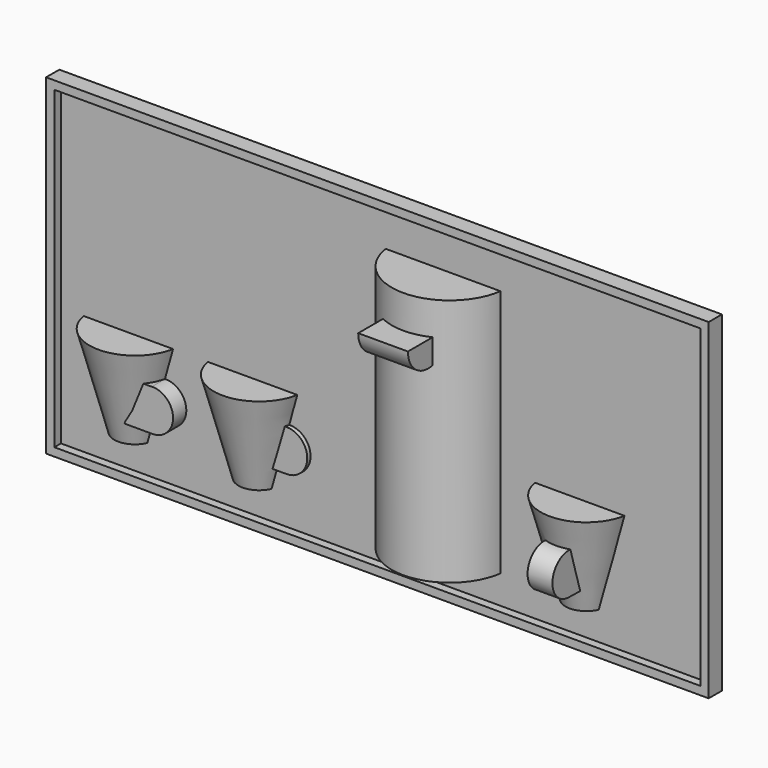
from build123d import *

# Parameters (mm, degrees)
F1_R      = 70
F2_DEPTH  = 300
F3_R      = 25
F4_R      = 55
F6_R      = 25
F7_R      = 55
F9_R      = 25
F10_R     = 55
F14_DEPTH = 30
F17_DEPTH = 15
F19_DEPTH = 15
F21_DEPTH = 30
F22_W     = 800
F22_H     = 400
F24_DEPTH = 20
F25_T     = -10


# Not quite as in the source:
# - a feature names something its author has since deleted; it is built from what else it names


with BuildPart() as f2:
    # F1 (on Top) → F2 (new body)
    with BuildSketch(Plane.XY):
        with Locations((70, 0)):
            Circle(F1_R)
    extrude(amount=F2_DEPTH)

    # F13 (on offset) → F14 (join, symmetric)
    with BuildSketch(Plane.YZ.offset(70)):
        with BuildLine():
            Line((-39.4232119037, 259.9333557068), (-100.5767880963, 259.9333557068))
            ThreePointArc((-100.5767880963, 259.9333557068), (-70, 229.4231392758), (-39.4232119037, 259.9333557068))
        make_face()
    extrude(amount=F14_DEPTH, both=True)


with BuildPart() as f5:
    # F3 (on Top) → F5 section 0
    with BuildSketch(Plane.XY):
        with Locations((235, 0)):
            Circle(F3_R)
    # F4 (on offset) → F5 section 1
    with BuildSketch(Plane.XY.offset(110)):
        with Locations((235, 0)):
            Circle(F4_R)
    loft()

    # F16 (on offset) → F17 (join, symmetric)
    with BuildSketch(Plane.YZ.offset(235)):
        with BuildLine():
            Line((-13.6413012409, 73.7935081125), (-44.023681798, 74.9809287811))
            ThreePointArc((-44.023681798, 74.9809287811), (-69.9889457828, 50.7433630762), (-45.5103433285, 25.005209549))
            Line((-45.5103433285, 25.005209549), (-13.6413012409, 24.3545078339))
            Line((-13.6413012409, 24.3545078339), (-13.6413012409, 73.7935081125))
        make_face()
    extrude(amount=F17_DEPTH, both=True)


with BuildPart() as f8:
    # F6 (on Top) → F8 section 0
    with BuildSketch(Plane.XY):
        with Locations((-160, 0)):
            Circle(F6_R)
    # F7 (on offset) → F8 section 1
    with BuildSketch(Plane.XY.offset(110)):
        with Locations((-160, 0)):
            Circle(F7_R)
    loft()

    # F18 (on Front) → F19 (join, symmetric)
    with BuildSketch(Plane.XZ):
        with BuildLine():
            Line((-153.4072975938, 25.0156882073), (-115.885530489, 25.0156882073))
            ThreePointArc((-115.885530489, 25.0156882073), (-90.0050194353, 49.4990543238), (-114.8837577761, 74.9997297534))
            Line((-114.8837577761, 74.9997297534), (-153.4072975938, 75.1788541675))
            Line((-153.4072975938, 75.1788541675), (-153.4072975938, 25.0156882073))
        make_face()
    extrude(amount=F19_DEPTH, both=True)


with BuildPart() as f11:
    # F9 (on Top) → F11 section 0
    with BuildSketch(Plane.XY):
        with Locations((-310, 0)):
            Circle(F9_R)
    # F10 (on offset) → F11 section 1
    with BuildSketch(Plane.XY.offset(110)):
        with Locations((-310, 0)):
            Circle(F10_R)
    loft()


with BuildPart() as f21:
    # F20 (on Front) → F21 (new body)
    with BuildSketch(Plane.XZ):
        with BuildLine():
            Line((-264.7419169597, 25.0013321726), (-265.2580830403, 25.0013321726))
            ThreePointArc((-265.2580830403, 25.0013321726), (-265, 25), (-264.7419169597, 25.0013321726))
        make_face()
        with BuildLine():
            Line((-307.4041914523, 25.0013321726), (-265.2580830403, 25.0013321726))
            Line((-265.2580830403, 25.0013321726), (-264.7419169597, 25.0013321726))
            ThreePointArc((-264.7419169597, 25.0013321726), (-240.0038230126, 50.4371910495), (-265.6162766145, 74.9924029084))
            Line((-265.6162766145, 74.9924029084), (-307.4041914523, 73.9619731903))
            Line((-307.4041914523, 73.9619731903), (-307.4041914523, 25.0013321726))
        make_face()
    extrude(amount=F21_DEPTH)


with BuildPart() as f24:
    # F22 (on Front) → F24 (new body)
    with BuildSketch(Plane.XZ):
        with Locations((-1.331, 155.6396274999)):
            Rectangle(F22_W, F22_H)
    extrude(amount=F24_DEPTH)

    # F25
    f25_openings = [f24.faces().sort_by_distance(p)[0] for p in [
        (-1.331, -20, 155.639627),
    ]]
    offset(amount=F25_T, openings=f25_openings)


solid = Compound([f2.part, f5.part, f8.part, f11.part, f21.part, f24.part])
